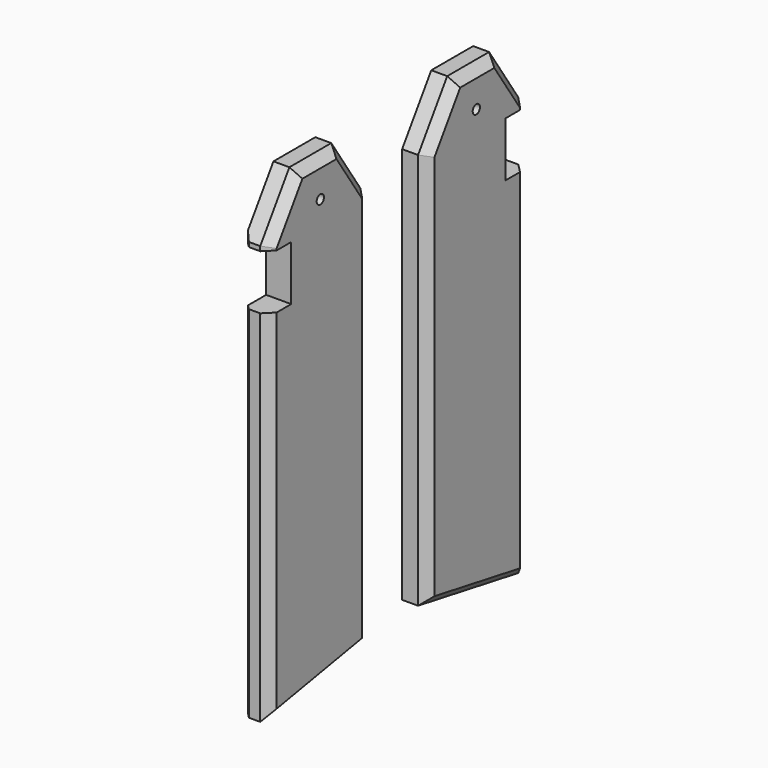
from build123d import *

# Parameters (mm, degrees)
F0_R      = 3.175
F1_DEPTH  = 17.4625
F2_SIZE   = 6.35
F2_2_SIZE = 6.35
F3_SIZE   = 3.175
F3_2_SIZE = 3.175


# Not quite as in the source:
# - a feature names something its author has since deleted; it is built from what else it names


with BuildPart() as f1:
    # F0 (on Right) → F1 (new body)
    with BuildSketch(Plane.YZ):
        Polygon((0, -314.8044504969), (0, -38.1), (-25.4, 0), (-61.9125, 0), (-87.3125, -38.1), (-87.3125, -41.275), (-68.2625, -41.275), (-68.2625, -79.375), (-87.3125, -79.375), (-87.3125, -330.2), align=None)
        with Locations((-42.8625, -25.4)):
            Circle(F0_R, mode=Mode.SUBTRACT)
    extrude(amount=F1_DEPTH)

    # F2
    f2_edges = [f1.edges().sort_by_distance(p)[0] for p in [
        (17.4625, -74.6125, -19.05),
        (17.4625, -43.65625, 0),
        (17.4625, -12.7, -19.05),
        (17.4625, 0, -176.452225),
        (17.4625, -87.3125, -39.6875),
        (17.4625, -43.65625, -322.502225),
        (17.4625, -87.3125, -204.7875),
    ]]
    chamfer(f2_edges, length=F2_SIZE)

    # F3#2
    f3_2_edges = [f1.edges().sort_by_distance(p)[0] for p in [
        (0, -87.3125, -39.6875),
        (0, -87.3125, -204.7875),
    ]]
    chamfer(f3_2_edges, length=F3_2_SIZE)


with BuildPart() as f1b:
    # F0 (on Right) → F1, piece 2 (new body)
    with BuildSketch(Plane.YZ):
        Polygon((137.5715984106, -38.1), (112.1715984106, 0), (75.6590984106, 0), (50.2590984106, -38.1), (50.2590984106, -314.8044504969), (137.5715984106, -330.2), (137.5715984106, -79.375), (118.5215984106, -79.375), (118.5215984106, -41.275), (137.5715984106, -41.275), align=None)
        with Locations((93.1215984106, -25.4)):
            Circle(F0_R, mode=Mode.SUBTRACT)
    extrude(amount=F1_DEPTH)

    # F2#2
    f2_2_edges = [f1b.edges().sort_by_distance(p)[0] for p in [
        (17.4625, 93.915348, -322.502225),
        (17.4625, 50.259098, -176.452225),
        (17.4625, 124.871598, -19.05),
        (17.4625, 93.915348, 0),
        (17.4625, 62.959098, -19.05),
        (17.4625, 137.571598, -204.7875),
        (17.4625, 137.571598, -39.6875),
    ]]
    chamfer(f2_2_edges, length=F2_2_SIZE)

    # F3
    f3_edges = [f1b.edges().sort_by_distance(p)[0] for p in [
        (0, 137.571598, -204.7875),
        (0, 137.571598, -39.6875),
    ]]
    chamfer(f3_edges, length=F3_SIZE)


solid = Compound([f1.part, f1b.part])
